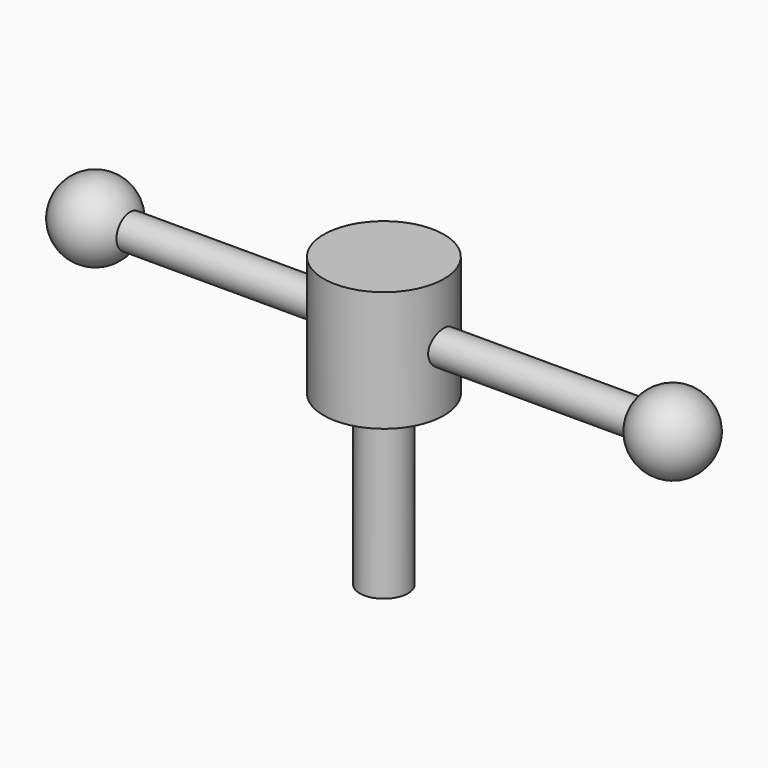
from build123d import *

# Parameters (mm, degrees)
F0_R     = 15.875
F0_R_2   = 6.35
F1_DEPTH = 31.75
F2_DEPTH = 44.45
F3_R     = 4.445
F4_DEPTH = 69.85


with BuildPart() as f1:
    # F0 (on Top) → F1 (new body)
    with BuildSketch(Plane.XY):
        Circle(F0_R)
        Circle(F0_R_2, mode=Mode.SUBTRACT)
        Circle(F0_R_2)
    extrude(amount=F1_DEPTH)

    # F0 (on Top) → F2 (join)
    with BuildSketch(Plane.XY):
        Circle(F0_R_2)
    extrude(amount=-F2_DEPTH)

    # F3 (on Right) → F4 (join, symmetric)
    with BuildSketch(Plane.YZ):
        with Locations((0, 15.875)):
            Circle(F3_R)
    extrude(amount=F4_DEPTH, both=True)

    # F5 (on Front) → F6 (revolve)
    with BuildSketch(Plane.XZ):
        with BuildLine():
            Line((76.2297678181, 15.875), (86.3897678181, 15.875))
            ThreePointArc((86.3897678181, 15.875), (78.5104738527, 25.7757060346), (67.0937087662, 20.32))
            Line((67.0937087662, 20.32), (69.85, 20.32))
            Line((69.85, 20.32), (69.85, 15.875))
            Line((69.85, 15.875), (76.2297678181, 15.875))
        make_face()
        with BuildLine():
            Line((-69.85, 15.875), (-66.0102321819, 15.875))
            ThreePointArc((-66.0102321819, 15.875), (-66.2695261473, 18.1557060346), (-67.03417313, 20.32))
            Line((-67.03417313, 20.32), (-69.85, 20.32))
            Line((-69.85, 20.32), (-69.85, 15.875))
        make_face()
        with BuildLine():
            Line((-69.85, 20.32), (-67.03417313, 20.32))
            ThreePointArc((-67.03417313, 20.32), (-78.4509382165, 25.7757060346), (-86.3302321819, 15.875))
            Line((-86.3302321819, 15.875), (-69.85, 15.875))
            Line((-69.85, 15.875), (-69.85, 20.32))
        make_face()
    revolve(axis=Axis((-81.717704612, 0, 15.875), (-1, 0, 0)))


solid = f1.part
